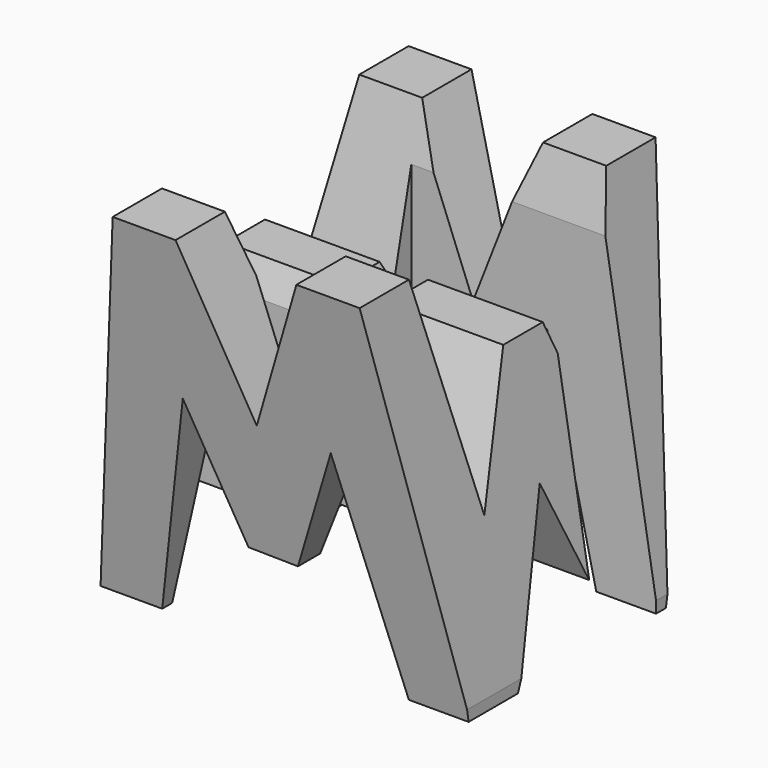
from build123d import *

# Parameters (mm, degrees)
F0_W      = 37.9036115915
F0_H      = 38.1
F1_DEPTH  = 38.1
F6_DEPTH  = 38.1
F8_DEPTH  = 38.1
F9_W      = 25.4
F9_H      = 7.62
F10_DEPTH = 38.1


# Not quite as in the source:
# - a feature names something its author has since deleted; it is built from what else it names


with BuildPart() as f1:
    # F0 (on Front) → F1 (new body)
    with BuildSketch(Plane.XZ):
        with Locations((18.9518057957, 19.05)):
            Rectangle(F0_W, F0_H)
    extrude(amount=F1_DEPTH)

    # F5 (on offset) → F6 (cut)
    with BuildSketch(Plane.YZ.offset(38.1)):
        Polygon((-6.35, 38.1), (-31.75, 38.1), (-26.67, 15.875), (-21.59, 28.575), (-16.51, 28.575), (-11.43, 15.875), align=None)
        Polygon((-31.75, 0), (-38.1, 38.1), (-38.1, 0), align=None)
        Polygon((-19.5393956542, 15.875), (-25.4, 0), (-12.7, 0), align=None)
        Polygon((0, 0), (0, 38.1), (-6.35, 0), align=None)
    extrude(amount=-F6_DEPTH, mode=Mode.SUBTRACT)

    # F7 (on offset) → F8 (cut)
    with BuildSketch(Plane.XZ.offset(38.1)):
        Polygon((25.2844232855, 38.196389037), (12.7511301009, 38.2289945719), (19.05, 22.225), align=None)
        Polygon((11.43, 22.225), (6.35, 0), (31.75, 0), (26.67, 22.225), (21.589256481, 9.4380885469), (16.51, 9.525), align=None)
        Polygon((38.1, 38.1630491376), (31.7472500896, 38.179575904), (31.75, 38.1630491376), (38.1, 0), align=None)
        Polygon((6.35, 38.2456472001), (0, 38.2621668126), (0, 0), align=None)
    extrude(amount=-F8_DEPTH, mode=Mode.SUBTRACT)

    # F9 (on offset) → F10 (cut)
    with BuildSketch(Plane.XY.offset(38.1)):
        with Locations((25.4, -11.43)):
            Rectangle(F9_W, F9_H)
        with Locations((12.7, -26.6583908668)):
            Rectangle(F9_W, F9_H)
    extrude(amount=-F10_DEPTH, mode=Mode.SUBTRACT)


solid = f1.part
